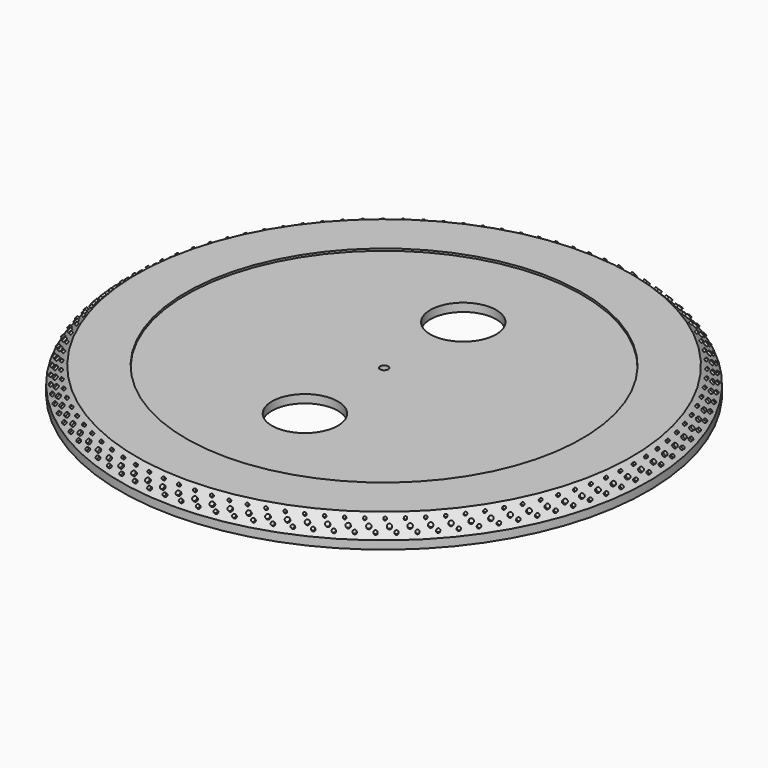
from build123d import *

# Parameters (mm, degrees)
F4_R      = 1.5875
F4_R_2    = 1.27
F4_R_3    = 1.016
F6_COUNT  = 100
F9_R      = 25.4
F10_DEPTH = 6.35
F11_R     = 3.175
F12_DEPTH = 6.35


with BuildPart() as f1:
    # F0 (on Right) → F1 (revolve)
    with BuildSketch(Plane.YZ):
        Polygon((0, 0), (0, 6.35), (-152.4, 6.35), (-152.4, 7.9375), (-190.5, 7.9375), (-203.2, -4.7625), (-203.2, -11.1125), (-177.8, -11.1125), (-177.8, 0), align=None)
    revolve(axis=Axis((0, 0, 1.1339256659), (0, 0, -1)))

    # F4 (on face) → F5 (join, up to the next surface of F1)
    with BuildSketch(Plane(origin=(0, -105.9539420908, 105.9539420908), x_dir=(-1, 0, 0), z_dir=(0, 0.7071067812, -0.7071067812))):
        with Locations((0, -138.6161817404)):
            Circle(F4_R)
        with Locations((-4.191, -142.4261817404)):
            Circle(F4_R_2)
        with Locations((2.54, -133.5361817404)):
            Circle(F4_R_3)
    f5 = extrude(until=Until.NEXT)

    # F6: F5 ×100 about axis
    f6_axis = Axis((0, 0, 1.1339256659), (0, 0, -1))
    for i in range(1, F6_COUNT):
        add(f5.rotate(f6_axis, i * 360 / F6_COUNT))

    # F7 (on Right) → F8 (revolve, cut)
    with BuildSketch(Plane.YZ):
        Polygon((-205.4450640303, -4.7625), (-192.7450640303, 7.9375), (-192.7450640303, 30.201989885), (-219.809487462, 30.201989885), (-219.809487462, -4.7625), align=None)
    revolve(axis=Axis((0, 0, 1.1339256659), (0, 0, -1)), mode=Mode.SUBTRACT)

    # F9 (on face) → F10 (cut, through all)
    with BuildSketch(Plane.XY.offset(6.35)):
        with Locations((0, 76.2)):
            Circle(F9_R)
        with Locations((0, -76.2)):
            Circle(F9_R)
    extrude(amount=-F10_DEPTH, mode=Mode.SUBTRACT)

    # F11 (on face) → F12 (cut, through all)
    with BuildSketch(Plane.XY.offset(6.35)):
        Circle(F11_R)
    extrude(amount=-F12_DEPTH, mode=Mode.SUBTRACT)


solid = f1.part
